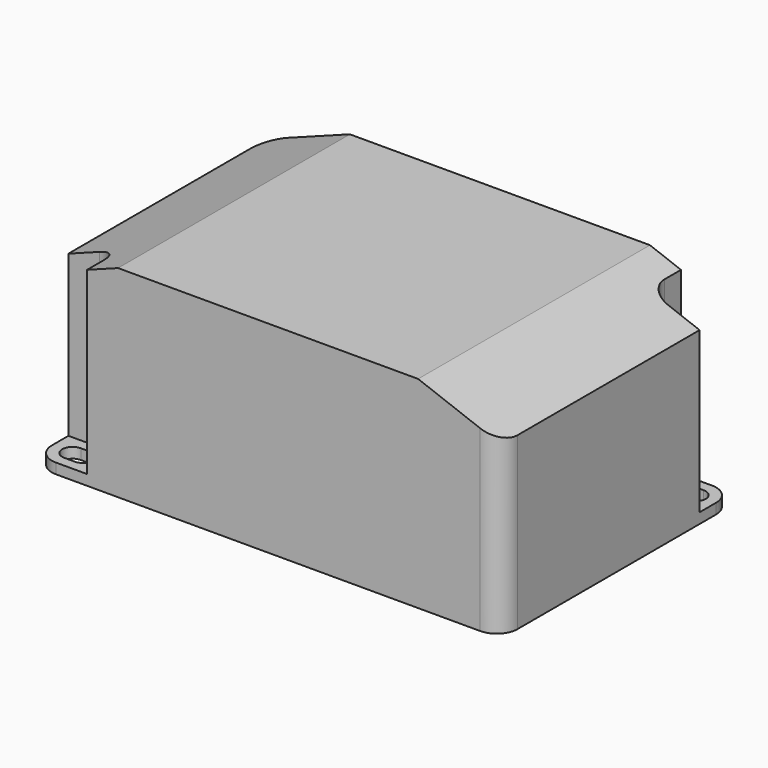
from build123d import *

# Parameters (mm, degrees)
F0_W        = 5
F0_H        = 4
F1_DEPTH    = 19.5
F2_T1_DEPTH = 69.5019292892
F3_START    = 1
F3_DEPTH    = 24
F4_R        = 2


# Not quite as in the source:
# - a fillet or chamfer that OpenCascade refuses, or shapes differently, is made with other operations: its cross-section is extruded or revolved along the edge and cut away or added


with BuildPart() as f1:
    # F0 (on Top) → F1 (new body)
    with BuildSketch(Plane.XY):
        Polygon((17.5, 14), (-22.5, 14), (-22.5, -10), (-17.5, -10), (-17.5, -14), (22.5, -14), (22.5, 10), (17.5, 10), align=None)
        with Locations((20, 12)):
            Rectangle(F0_W, F0_H)
        with BuildLine():
            ThreePointArc((19.5, 11), (18.5, 12), (19.5, 13))
            Line((19.5, 13), (20.5, 13))
            ThreePointArc((20.5, 13), (21.5, 12), (20.5, 11))
            Line((20.5, 11), (19.5, 11))
        make_face(mode=Mode.SUBTRACT)
        with Locations((-20, -12)):
            Rectangle(F0_W, F0_H)
        with BuildLine():
            ThreePointArc((-20.5, -13), (-21.5, -12), (-20.5, -11))
            Line((-20.5, -11), (-19.5, -11))
            ThreePointArc((-19.5, -11), (-18.5, -12), (-19.5, -13))
            Line((-19.5, -13), (-20.5, -13))
        make_face(mode=Mode.SUBTRACT)
    extrude(amount=F1_DEPTH)

    # F2: chamfer of 3 x 8 on 2 edges, made by hand

    # F2_s2 → F2_t1 (cut)
    with BuildSketch(Plane.XZ.offset(-34.7509646446)):
        Polygon((-22.5, 16.5), (-14.5, 19.5), (-22.5, 19.5), align=None)
        Polygon((22.5, 16.5), (14.5, 19.5), (22.5, 19.5), align=None)
    extrude(amount=F2_T1_DEPTH, mode=Mode.SUBTRACT)

    # F0 (on Top) → F3 (cut)
    with BuildSketch(Plane.XY.offset(F3_START)):
        with Locations((-20, -12)):
            Rectangle(F0_W, F0_H)
        with BuildLine():
            ThreePointArc((-20.5, -13), (-21.5, -12), (-20.5, -11))
            Line((-20.5, -11), (-19.5, -11))
            ThreePointArc((-19.5, -11), (-18.5, -12), (-19.5, -13))
            Line((-19.5, -13), (-20.5, -13))
        make_face(mode=Mode.SUBTRACT)
        with Locations((20, 12)):
            Rectangle(F0_W, F0_H)
        with BuildLine():
            ThreePointArc((19.5, 11), (18.5, 12), (19.5, 13))
            Line((19.5, 13), (20.5, 13))
            ThreePointArc((20.5, 13), (21.5, 12), (20.5, 11))
            Line((20.5, 11), (19.5, 11))
        make_face(mode=Mode.SUBTRACT)
    extrude(amount=F3_DEPTH, mode=Mode.SUBTRACT)

    # F4
    f4_edges = [f1.edges().sort_by_distance(p)[0] for p in [
        (-17.5, -10, 9.6875),
        (17.5, 10, 9.6875),
        (22.5, -14, 8.25),
        (22.5, 14, 0.5),
        (-22.5, 14, 8.25),
        (-22.5, -14, 0.5),
    ]]
    fillet(f4_edges, radius=F4_R)


solid = f1.part
